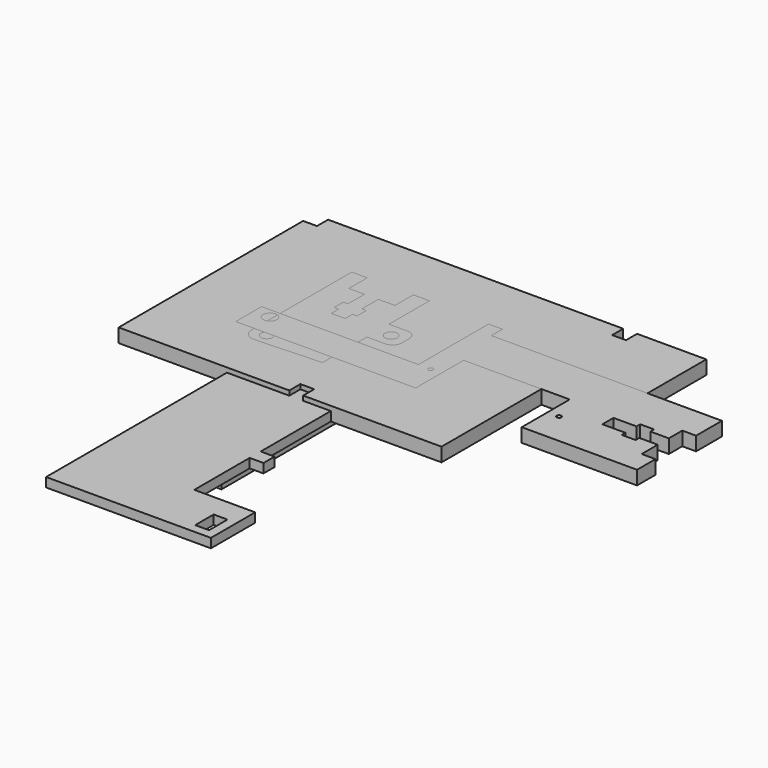
from build123d import *

# Parameters (mm, degrees)
F0_W     = 13.2
F0_H     = 12
F0_W_2   = 3
F0_H_2   = 5
F0_H_3   = 3
F0_W_3   = 3.2
F0_H_4   = 3.2
F1_DEPTH = 2
F3_DEPTH = 3
F4_R     = 0.5
F4_W     = 12
F4_H     = 23
F4_H_2   = 22
F5_DEPTH = 3
F6_R     = 1.35
F6_R_2   = 1.25
F7_DEPTH = 3
F8_W     = 3
F8_H     = 3
F8_R     = 1.5
F8_R_2   = 0.5
F9_DEPTH = 3


with BuildPart() as f1:
    # F0 (on Top) → F1 (new body)
    with BuildSketch(Plane.XY):
        Polygon((-3.4e-09, -18.5), (-5.1, -18.5), (-11.533, -18.5), (-11.533, -75.5), (11, -75.5), (11, -63.5), (11, -48.5), (11, -45.5), (11, -18.5), (5.1, -18.5), align=None)
        with Locations((17.6, -69.5)):
            Rectangle(F0_W, F0_H)
        with Locations((20.7, -71)):
            Rectangle(F0_W_2, F0_H_2, mode=Mode.SUBTRACT)
        with Locations((12.5, -47)):
            Rectangle(F0_W_2, F0_H_3)
        Polygon((11, 14.3), (11, 17.5), (-11, 17.5), (-11, -17.5), (-5.1, -17.5), (-5.1, -16.5), (0, -16.5), (5.1, -16.5), (5.1, -17.5), (11, -17.5), align=None)
        with Locations((12.6, 15.9)):
            Rectangle(F0_W_3, F0_H_4)
        with BuildLine():
            Line((5.1, -18.5), (5.1, -17.5))
            Line((5.1, -17.5), (1, -17.5))
            ThreePointArc((1, -17.5), (0.70710678, -18.2071067824), (-3.4e-09, -18.5))
            Line((-3.4e-09, -18.5), (5.1, -18.5))
        make_face()
        with BuildLine():
            Line((1, -17.5), (5.1, -17.5))
            Line((5.1, -17.5), (5.1, -16.5))
            Line((5.1, -16.5), (0, -16.5))
            ThreePointArc((0, -16.5), (0.7071067812, -16.7928932188), (1, -17.5))
        make_face()
        with BuildLine():
            Line((-1, -17.5), (-5.1, -17.5))
            Line((-5.1, -17.5), (-5.1, -18.5))
            Line((-5.1, -18.5), (-3.4e-09, -18.5))
            ThreePointArc((-3.4e-09, -18.5), (-0.7071067824, -18.20710678), (-1, -17.5))
        make_face()
        with BuildLine():
            Line((-5.1, -16.5), (-5.1, -17.5))
            Line((-5.1, -17.5), (-1, -17.5))
            ThreePointArc((-1, -17.5), (-0.7071067812, -16.7928932188), (0, -16.5))
            Line((0, -16.5), (-5.1, -16.5))
        make_face()
    extrude(amount=F1_DEPTH)


with BuildPart() as f3:
    # F2 (on Top) → F3 (new body)
    with BuildSketch(Plane.XY):
        Polygon((50, 26.5), (35, 26.5), (35, 23.5), (35, 7.5), (50, 7.5), align=None)
        Polygon((32, 23.5), (32, 26.5), (-32, 26.5), (-32, 23.5), (-35, 23.5), (-35, -26.5), (2, -26.5), (2, -23.5), (5, -23.5), (5, -26.5), (35, -26.5), (35, 7.5), (35, 23.5), align=None)
    extrude(amount=F3_DEPTH)


with BuildPart() as f5:
    # F4 (on Top) → F5 (new body)
    with BuildSketch(Plane.XY):
        Polygon((8.5, -17), (8.5, 17), (-8.5, 17), (-8.5, -17), (-5.5, -17), (0, -17), (4.5, -17), align=None)
        with Locations((0, -14)):
            Circle(F4_R, mode=Mode.SUBTRACT)
        with Locations((0, -0.5)):
            Rectangle(F4_W, F4_H, mode=Mode.SUBTRACT)
        with Locations((0, 13)):
            Circle(F4_R, mode=Mode.SUBTRACT)
        with BuildLine():
            Line((4.5, -19), (4.5, -17))
            Line((4.5, -17), (0, -17))
            ThreePointArc((0, -17), (0.7071067812, -17.2928932188), (1, -18))
            ThreePointArc((1, -18), (0.70710678, -18.7071067824), (-3.4e-09, -19))
            Line((-3.4e-09, -19), (4.5, -19))
        make_face()
        with BuildLine():
            Line((0, -17), (-5.5, -17))
            Line((-5.5, -17), (-5.5, -19))
            Line((-5.5, -19), (-3.4e-09, -19))
            ThreePointArc((-3.4e-09, -19), (-1, -17.9999999983), (0, -17))
        make_face()
        Polygon((8.5, -19), (4.5, -19), (-3.4e-09, -19), (-5.5, -19), (-8.5, -19), (-8.5, -53), (8.5, -53), align=None)
        with Locations((-0.0608968027, -36)):
            Rectangle(F4_W, F4_H_2, mode=Mode.SUBTRACT)
        with Locations((0, -49.5)):
            Circle(F4_R, mode=Mode.SUBTRACT)
        with Locations((0, -22.5)):
            Circle(F4_R, mode=Mode.SUBTRACT)
    extrude(amount=-F5_DEPTH)


with BuildPart() as f7:
    # F6 (on Top) → F7 (new body)
    with BuildSketch(Plane.XY):
        with BuildLine():
            Line((4, 3), (0, 3))
            Line((0, 3), (0, -3))
            Line((0, -3), (4, -3))
            ThreePointArc((4, -3), (5.4142135624, -2.4142135624), (6, -1))
            Line((6, -1), (6, 1))
            ThreePointArc((6, 1), (5.4142135624, 2.4142135624), (4, 3))
        make_face()
        with Locations((2.8909749817, 0)):
            Circle(F6_R, mode=Mode.SUBTRACT)
        with BuildLine():
            Line((-13.5, 14), (-16.8499713292, 14))
            Line((-16.8499713292, 14), (-16.8499713292, -13.1433860515))
            ThreePointArc((-16.8499713292, -13.1433860515), (-15.9964054633, -15.0246767366), (-14.0185676156, -15.6213230117))
            Line((-14.0185676156, -15.6213230117), (0, -15))
            Line((0, -15), (0, -13.7464547476))
            Line((0, -13.7464547476), (0, -3))
            Line((0, -3), (0, 3))
            Line((0, 3), (0, 14))
            Line((0, 14), (-3.5, 14))
            Line((-3.5, 14), (-3.5, 9))
            Line((-3.5, 9), (-7.1, 9))
            Line((-7.1, 9), (-7.1, 4.5))
            Line((-7.1, 4.5), (-6.1, 4.5))
            Line((-6.1, 4.5), (-6.1, 2))
            Line((-6.1, 2), (-7.1, 2))
            Line((-7.1, 2), (-7.1, 0))
            Line((-7.1, 0), (-10.1, 0))
            Line((-10.1, 0), (-10.1, 2))
            Line((-10.1, 2), (-11.1, 2))
            Line((-11.1, 2), (-11.1, 4.5))
            Line((-11.1, 4.5), (-10.1, 4.5))
            Line((-10.1, 4.5), (-10.1, 9))
            Line((-10.1, 9), (-13.5, 9))
            Line((-13.5, 9), (-13.5, 14))
        make_face()
        with Locations((-13.5999713292, -13.1433860515)):
            Circle(F6_R_2, mode=Mode.SUBTRACT)
    extrude(amount=F7_DEPTH)


with BuildPart() as f9:
    # F8 (on Top) → F9 (new body)
    with BuildSketch(Plane.XY):
        with Locations((14.6363672018, 12.071258156)):
            Rectangle(F8_W, F8_H)
        with BuildLine():
            Line((13.1363672018, -5.428741844), (-20.8636327982, -5.428741844))
            Line((-20.8636327982, -5.428741844), (-20.8636327982, -12.428741844))
            Line((-20.8636327982, -12.428741844), (18.1363672018, -12.428741844))
            Line((18.1363672018, -12.428741844), (18.1363672018, -5.428741844))
            Line((18.1363672018, -5.428741844), (16.3363672018, -5.428741844))
            ThreePointArc((16.3363672018, -5.428741844), (15.8363672018, -5.928741844), (15.3363672018, -5.428741844))
            Line((15.3363672018, -5.428741844), (13.1363672018, -5.428741844))
        make_face()
        with Locations((-17.3636327982, -7.528741844)):
            Circle(F8_R, mode=Mode.SUBTRACT)
        with BuildLine():
            Line((13.1363672018, 10.571258156), (13.1363672018, -5.428741844))
            Line((13.1363672018, -5.428741844), (15.3363672018, -5.428741844))
            ThreePointArc((15.3363672018, -5.428741844), (15.8363672018, -4.928741844), (16.3363672018, -5.428741844))
            Line((16.3363672018, -5.428741844), (18.1363672018, -5.428741844))
            Line((18.1363672018, -5.428741844), (18.1363672018, 0.571258156))
            Line((18.1363672018, 0.571258156), (18.1363672018, 10.571258156))
            Line((18.1363672018, 10.571258156), (16.1363672018, 10.571258156))
            Line((16.1363672018, 10.571258156), (13.1363672018, 10.571258156))
        make_face()
        Polygon((41.1363672018, 0.571258156), (41.1363672018, -12.428741844), (66.1363672018, -12.428741844), (66.1363672018, -7.428741844), (63.1363672018, -7.428741844), (63.1363672018, -3.0713211745), (59.1363672018, -3.0713211745), (59.1363672018, -4.0713211745), (56.1363672018, -4.0713211745), (56.1363672018, -3.0713211745), (51.1363672018, -3.0713211745), (51.1363672018, -0.0713211745), (56.1363672018, -0.0713211745), (56.1363672018, 0.9286788255), (59.1363672018, 0.9286788255), (59.1363672018, -0.0713211745), (63.1363672018, -0.0713211745), (63.1363672018, 3.571258156), (66.1363672018, 3.571258156), (66.1363672018, 10.571258156), (18.1363672018, 10.571258156), (18.1363672018, 0.571258156), align=None)
        with Locations((43.6363672018, -5.428741844)):
            Circle(F8_R_2, mode=Mode.SUBTRACT)
    extrude(amount=F9_DEPTH)


solid = Compound([f1.part, f3.part, f5.part, f7.part, f9.part])
